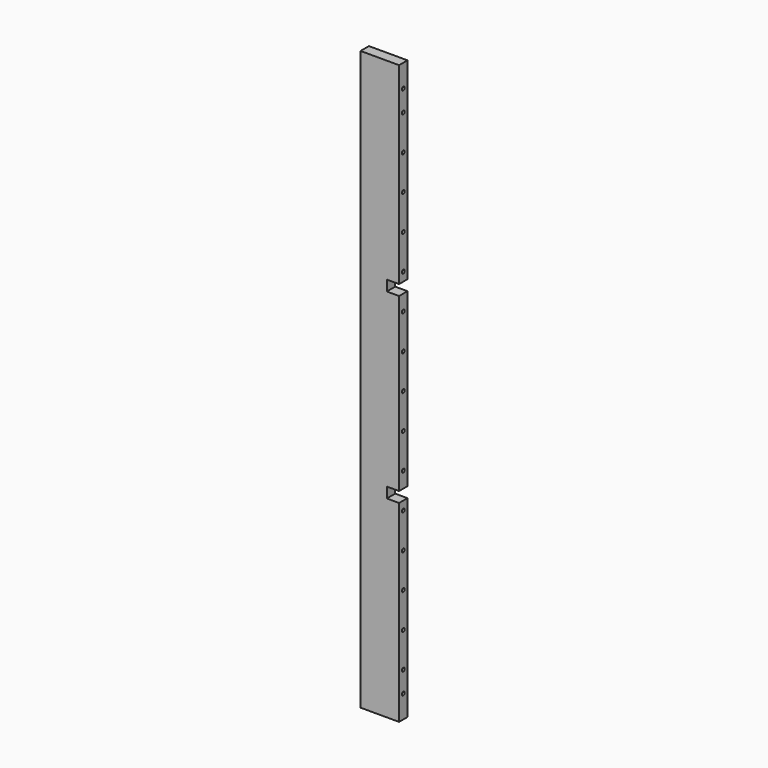
from build123d import *

# Parameters (mm, degrees)
F0_W     = 139.7
F0_H     = 38.1
F1_DEPTH = 2095.5
F2_R     = 6.35
F3_DEPTH = 152.4
F4_W     = 38.1
F4_H     = 38.1
F5_DEPTH = 44.45


with BuildPart() as f1:
    # F0 (on Top) → F1 (new body)
    with BuildSketch(Plane.XY):
        Rectangle(F0_W, F0_H)
    extrude(amount=F1_DEPTH)

    # F2 (on face) → F3 (cut)
    with BuildSketch(Plane(origin=(-69.85, 0, 0), x_dir=(0, -1, 0), z_dir=(-1, 0, 0))):
        with BuildLine():
            ThreePointArc((6.35, 1047.75), (0, 1054.1), (-6.35, 1047.75))
            Line((-6.35, 1047.75), (6.35, 1047.75))
        make_face()
        with BuildLine():
            Line((6.35, 1047.75), (-6.35, 1047.75))
            ThreePointArc((-6.35, 1047.75), (0, 1041.4), (6.35, 1047.75))
        make_face()
        with Locations((0, 1174.75)):
            Circle(F2_R)
        with Locations((0, 1301.75)):
            Circle(F2_R)
        with Locations((0, 1428.75)):
            Circle(F2_R)
        with Locations((0, 1555.75)):
            Circle(F2_R)
        with Locations((0, 1682.75)):
            Circle(F2_R)
        with Locations((0, 1809.75)):
            Circle(F2_R)
        with Locations((0, 1936.75)):
            Circle(F2_R)
        with Locations((0, 920.75)):
            Circle(F2_R)
        with Locations((0, 666.75)):
            Circle(F2_R)
        with Locations((0, 539.75)):
            Circle(F2_R)
        with Locations((0, 412.75)):
            Circle(F2_R)
        with Locations((0, 285.75)):
            Circle(F2_R)
        with Locations((0, 158.75)):
            Circle(F2_R)
        with Locations((0, 793.75)):
            Circle(F2_R)
        with Locations((0, 2012.95)):
            Circle(F2_R)
        with Locations((0, 82.55)):
            Circle(F2_R)
    extrude(amount=-F3_DEPTH, mode=Mode.SUBTRACT)

    # F4 (on face) → F5 (cut)
    with BuildSketch(Plane.YZ.offset(69.85)):
        with Locations((0, 717.55)):
            Rectangle(F4_W, F4_H)
        with Locations((0, 1377.95)):
            Rectangle(F4_W, F4_H)
    extrude(amount=-F5_DEPTH, mode=Mode.SUBTRACT)


solid = f1.part
